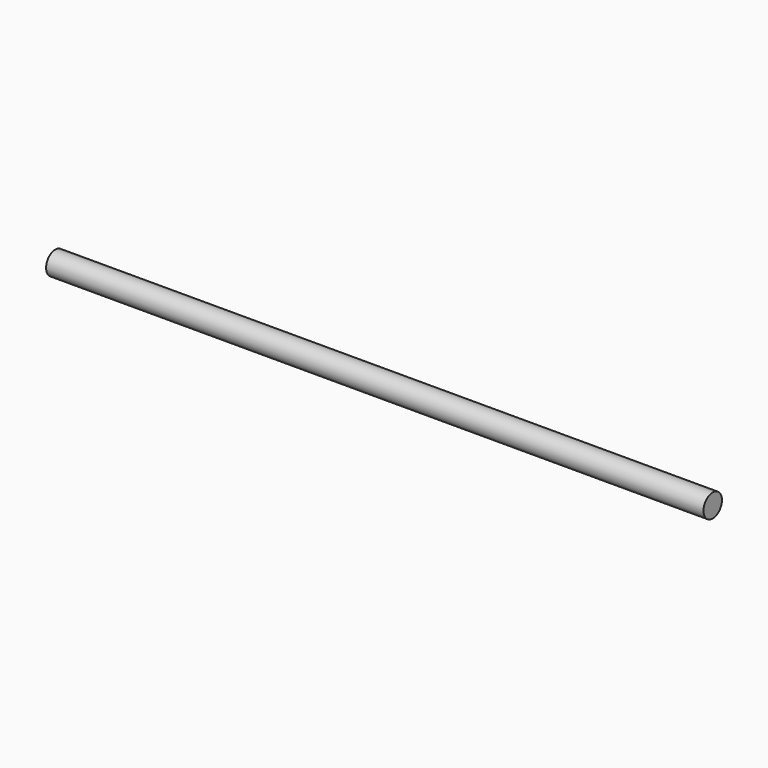
from build123d import *

# Parameters (mm, degrees)
F0_W = 72.4511221051
F0_H = 1.27


# Not quite as in the source:
# - a feature of the source that left no trace in its solid (it failed there, or was rolled back) is left out


with BuildPart() as f1:
    # F0 (on Top) → F1 (revolve)
    with BuildSketch(Plane.XY):
        with Locations((36.2255610526, -0.635)):
            Rectangle(F0_W, F0_H)
    revolve(axis=Axis((36.2255610526, 0, 0), (1, 0, 0)))


solid = f1.part
